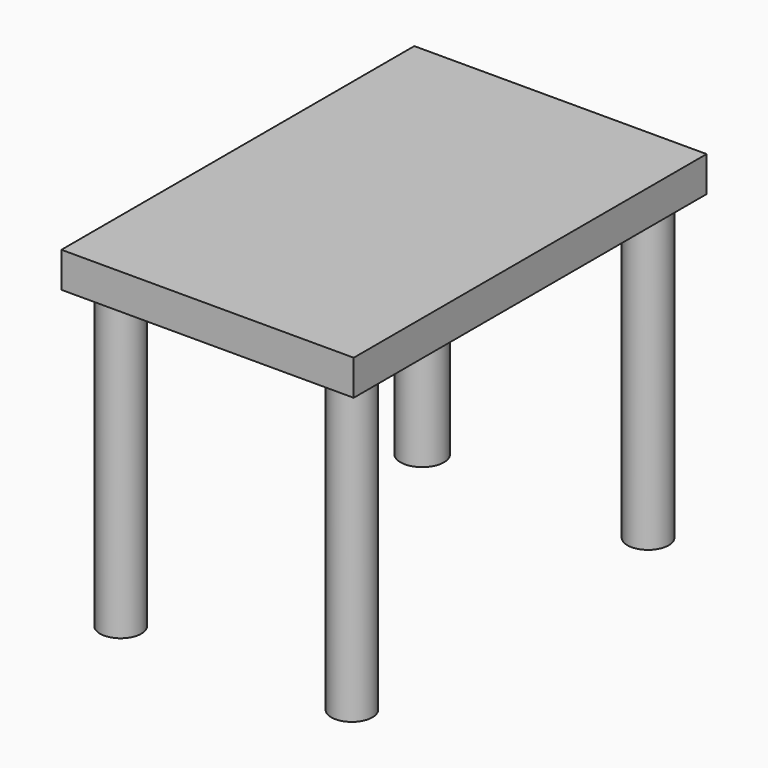
from build123d import *

# Parameters (mm, degrees)
F0_W     = 151.485607028
F0_H     = 18.2879995555
F1_DEPTH = 228.6
F2_T     = -2.54
F3_R     = 10.6799813772
F3_R_2   = 11.2854145599
F3_R_3   = 10.6922207588
F3_R_4   = 10.6551247764
F8_DEPTH = 170.18


# Not quite as in the source:
# - the program builds the solid bodies; features that only make, move or delete a surface that nothing else refers to are left out


with BuildPart() as f1:
    # F0 (on Front) → F1 (new body)
    with BuildSketch(Plane.XZ):
        with Locations((0, 9.1439997777)):
            Rectangle(F0_W, F0_H)
    extrude(amount=F1_DEPTH)

    # F2
    f2_openings = [f1.faces().sort_by_distance(p)[0] for p in [
        (0, -114.3, 0),
    ]]
    offset(amount=F2_T, openings=f2_openings)

    # F3 (on face) → F8 (join)
    with BuildSketch(Plane(origin=(0, 0, 15.7479995555), x_dir=(1, 0, 0), z_dir=(0, 0, -1))):
        with Locations((-58.2167990506, 212.1407985687)):
            Circle(F3_R)
        with Locations((-56.9975972176, 18.2879958302)):
            Circle(F3_R_2)
        with Locations((60.0456036627, 18.2879958302)):
            Circle(F3_R_3)
        with Locations((60.6552027166, 210.921600461)):
            Circle(F3_R_4)
    extrude(amount=F8_DEPTH)


solid = f1.part
